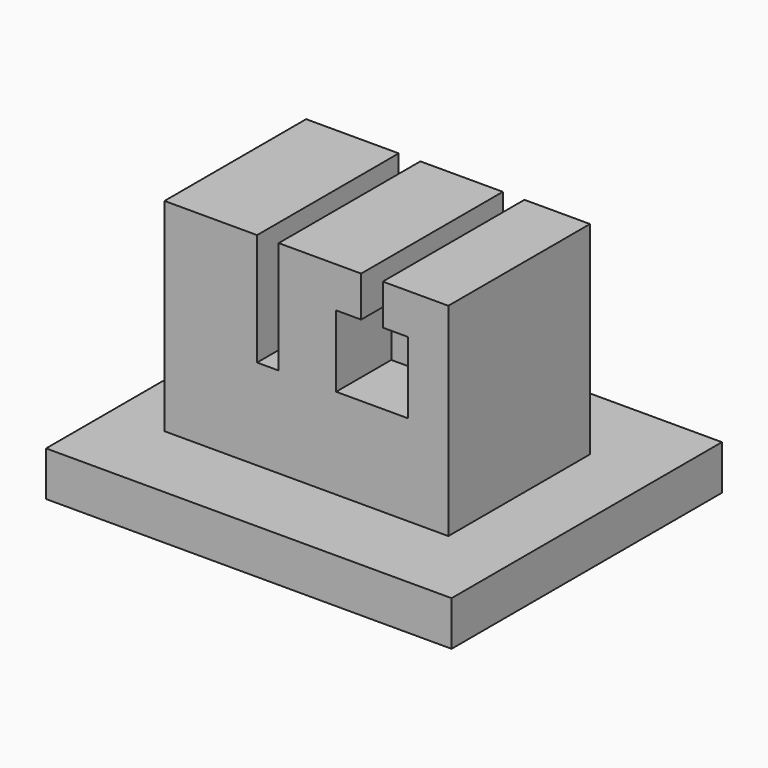
from build123d import *

# Parameters (mm, degrees)
F0_W      = 30
F0_H      = 25
F1_DEPTH  = 3.3
F2_W      = 21
F2_H      = 13.1
F3_DEPTH  = 15
F4_W      = 5.3
F4_H      = 5.3
F5_DEPTH  = 5.1
F6_W      = 1.6
F6_H      = 13.1
F7_DEPTH  = 8.3
F8_W      = 5.3
F8_H      = 5.3
F9_DEPTH  = 5.1
F10_W     = 1.6
F10_H     = 13.1
F11_DEPTH = 8.3


# Not quite as in the source:
# - a feature names something its author has since deleted; it is built from what else it names


with BuildPart() as f1:
    # F0 (on Top) → F1 (new body)
    with BuildSketch(Plane.XY):
        Rectangle(F0_W, F0_H)
    extrude(amount=F1_DEPTH)

    # F2 (on face) → F3 (join)
    with BuildSketch(Plane.XY.offset(3.3)):
        with Locations((-0.5, 0)):
            Rectangle(F2_W, F2_H)
    extrude(amount=F3_DEPTH)

    # F4 (on face) → F5 (cut)
    with BuildSketch(Plane.XZ.offset(6.55)):
        with Locations((4.35, 12.65)):
            Rectangle(F4_W, F4_H)
    extrude(amount=-F5_DEPTH, mode=Mode.SUBTRACT)

    # F6 (on face) → F7 (cut)
    with BuildSketch(Plane.XY.offset(18.3)):
        with Locations((4.35, 0)):
            Rectangle(F6_W, F6_H)
    extrude(amount=-F7_DEPTH, mode=Mode.SUBTRACT)

    # F8 (on face) → F9 (cut)
    with BuildSketch(Plane(origin=(0, 6.55, 0), x_dir=(-1, 0, 0), z_dir=(0, 1, 0))):
        with Locations((3.35, 12.65)):
            Rectangle(F8_W, F8_H)
    extrude(amount=-F9_DEPTH, mode=Mode.SUBTRACT)

    # F10 (on face) → F11 (cut)
    with BuildSketch(Plane.XY.offset(18.3)):
        with Locations((-3.35, 0)):
            Rectangle(F10_W, F10_H)
    extrude(amount=-F11_DEPTH, mode=Mode.SUBTRACT)


solid = f1.part
